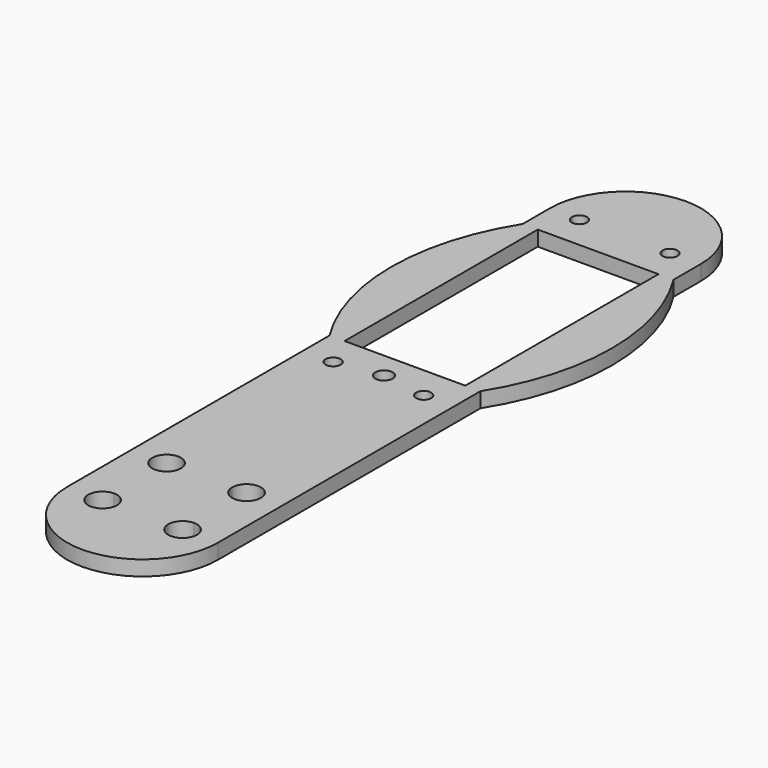
from build123d import *

# Parameters (mm, degrees)
F1_DEPTH = 2.54
F2_R     = 1.4605
F3_DEPTH = 2.541
F5_DEPTH = 2.54
F4_R     = 1.27
F6_DEPTH = 25.4


with BuildPart() as f1:
    # F0 (on Top) → F1 (new body)
    with BuildSketch(Plane.XY):
        with BuildLine():
            Line((12.7, -50.8), (12.7, 50.8))
            ThreePointArc((12.7, 50.8), (0, 63.5), (-12.7, 50.8))
            Line((-12.7, 50.8), (-12.7, -50.8))
            ThreePointArc((-12.7, -50.8), (0, -63.5), (12.7, -50.8))
        make_face()
        with BuildLine():
            Line((4.318, -50.7966617284), (-4.318, -50.7966617284))
            ThreePointArc((-4.318, -50.7966617284), (-8.437248663, -52.5029103914), (-6.731, -48.3836617284))
            Line((-6.731, -48.3836617284), (-6.731, -39.7476617284))
            ThreePointArc((-6.731, -39.7476617284), (-8.437248663, -35.6284130654), (-4.318, -37.3346617284))
            Line((-4.318, -37.3346617284), (4.318, -37.3346617284))
            ThreePointArc((4.318, -37.3346617284), (6.731, -34.9216617284), (9.144, -37.3346617284))
            ThreePointArc((9.144, -37.3346617284), (8.437248663, -39.0409103914), (6.731, -39.7476617284))
            Line((6.731, -39.7476617284), (6.731, -48.3836617284))
            ThreePointArc((6.731, -48.3836617284), (8.437248663, -49.0904130654), (9.144, -50.7966617284))
            ThreePointArc((9.144, -50.7966617284), (6.731, -53.2096617284), (4.318, -50.7966617284))
        make_face(mode=Mode.SUBTRACT)
        with BuildLine():
            ThreePointArc((-6.731, -48.3836617284), (-5.024751337, -49.0904130654), (-4.318, -50.7966617284))
            Line((-4.318, -50.7966617284), (4.318, -50.7966617284))
            ThreePointArc((4.318, -50.7966617284), (5.024751337, -49.0904130654), (6.731, -48.3836617284))
            Line((6.731, -48.3836617284), (6.731, -39.7476617284))
            ThreePointArc((6.731, -39.7476617284), (5.024751337, -39.0409103914), (4.318, -37.3346617284))
            Line((4.318, -37.3346617284), (-4.318, -37.3346617284))
            ThreePointArc((-4.318, -37.3346617284), (-5.024751337, -39.0409103914), (-6.731, -39.7476617284))
            Line((-6.731, -39.7476617284), (-6.731, -48.3836617284))
        make_face()
    extrude(amount=F1_DEPTH)

    # F2 (on face) → F3 (cut, through all)
    with BuildSketch(Plane.XY.offset(2.54)):
        Circle(F2_R)
    extrude(amount=-F3_DEPTH, mode=Mode.SUBTRACT)

    # F4 (on face) → F5 (join, through all)
    with BuildSketch(Plane.XY.offset(2.54)):
        with BuildLine():
            ThreePointArc((12.7, 4.4121561861), (18.5710130473, 24.7321561861), (12.7, 45.0521561861))
            Line((12.7, 45.0521561861), (12.7, 4.4121561861))
        make_face()
        with BuildLine():
            Line((-12.7, 4.4121561861), (-12.7, 45.0521561861))
            ThreePointArc((-12.7, 45.0521561861), (-18.5710130473, 24.7321561861), (-12.7, 4.4121561861))
        make_face()
    extrude(amount=-F5_DEPTH)

    # F4 (on face) → F6 (cut)
    with BuildSketch(Plane.XY.offset(2.54)):
        Polygon((10.16, 4.4121561861), (10.16, 45.0521561861), (7.62, 45.0521561861), (7.62, 37.1781561861), (0, 37.1781561861), (-7.62, 37.1781561861), (-7.62, 45.0521561861), (-10.16, 45.0521561861), (-10.16, 4.4121561861), align=None)
        Polygon((7.62, 37.1781561861), (7.62, 45.0521561861), (-7.62, 45.0521561861), (-7.62, 37.1781561861), (0, 37.1781561861), align=None)
        with BuildLine():
            ThreePointArc((6.35, 50.6401561861), (6.7219743879, 49.742130574), (7.62, 49.3701561861))
            Line((7.62, 49.3701561861), (7.62, 50.6401561861))
            Line((7.62, 50.6401561861), (6.35, 50.6401561861))
        make_face()
        with BuildLine():
            Line((7.62, 50.6401561861), (7.62, 49.3701561861))
            ThreePointArc((7.62, 49.3701561861), (8.5180256121, 49.742130574), (8.89, 50.6401561861))
            Line((8.89, 50.6401561861), (7.62, 50.6401561861))
        make_face()
        with BuildLine():
            Line((7.62, 50.6401561861), (8.89, 50.6401561861))
            ThreePointArc((8.89, 50.6401561861), (7.62, 51.9101561861), (6.35, 50.6401561861))
            Line((6.35, 50.6401561861), (7.62, 50.6401561861))
        make_face()
        with BuildLine():
            ThreePointArc((-8.89, 50.6401561861), (-8.5180256121, 49.742130574), (-7.62, 49.3701561861))
            Line((-7.62, 49.3701561861), (-7.62, 50.6401561861))
            Line((-7.62, 50.6401561861), (-8.89, 50.6401561861))
        make_face()
        with BuildLine():
            Line((-7.62, 50.6401561861), (-7.62, 49.3701561861))
            ThreePointArc((-7.62, 49.3701561861), (-6.7219743879, 49.742130574), (-6.35, 50.6401561861))
            Line((-6.35, 50.6401561861), (-7.62, 50.6401561861))
        make_face()
        with BuildLine():
            Line((-8.89, 50.6401561861), (-7.62, 50.6401561861))
            Line((-7.62, 50.6401561861), (-6.35, 50.6401561861))
            ThreePointArc((-6.35, 50.6401561861), (-7.62, 51.9101561861), (-8.89, 50.6401561861))
        make_face()
        with Locations((-7.62, -1.1758438139)):
            Circle(F4_R)
        with Locations((7.62, -1.1758438139)):
            Circle(F4_R)
    extrude(amount=-F6_DEPTH, mode=Mode.SUBTRACT)


solid = f1.part
